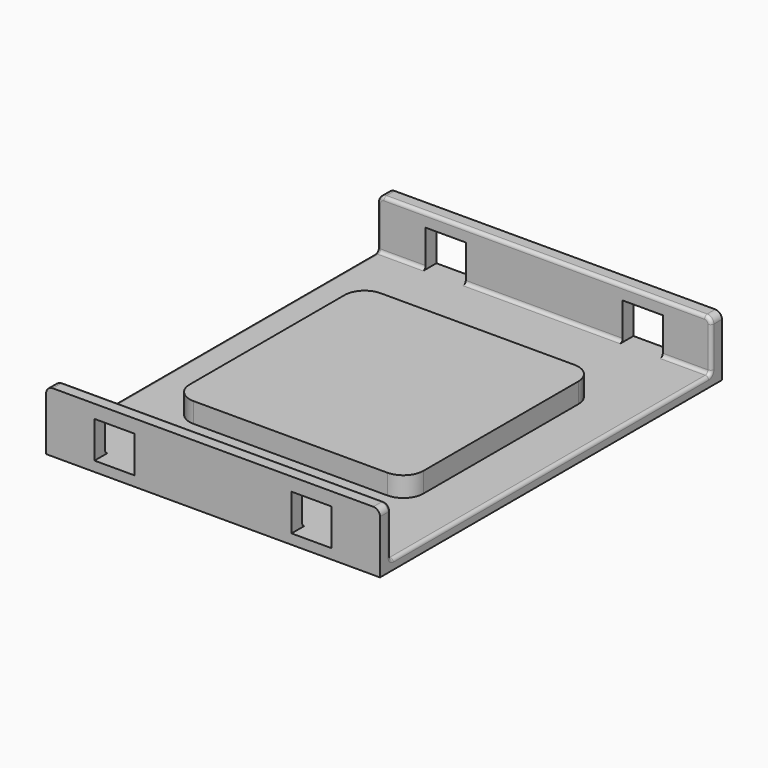
from build123d import *

# Parameters (mm, degrees)
F0_W      = 50
F0_H      = 60
F1_DEPTH  = 1.5
F2_W      = 20
F2_H      = 2
F3_DEPTH  = 9
F4_W      = 6
F4_H      = 5.5
F5_DEPTH  = 32
F6_W      = 35
F6_H      = 35
F7_DEPTH  = 4.5
F8_R      = 3
F9_DEPTH  = 5
F10_DEPTH = 5
F11_DEPTH = 5
F12_DEPTH = 5
F13_R     = 1
F14_R     = 0.5


with BuildPart() as f1:
    # F0 (on Top) → F1 (new body)
    with BuildSketch(Plane.XY):
        Rectangle(F0_W, F0_H)
    extrude(amount=F1_DEPTH)

    # F2 (on Top) → F3 (join)
    with BuildSketch(Plane.XY):
        with Locations((10, 31)):
            Rectangle(F2_W, F2_H)
        with Locations((-10, 31)):
            Rectangle(F2_W, F2_H)
        with Locations((-10, -31)):
            Rectangle(F2_W, F2_H)
        with Locations((10, -31)):
            Rectangle(F2_W, F2_H)
    extrude(amount=F3_DEPTH)

    # F4 (on Front) → F5 (cut, symmetric)
    with BuildSketch(Plane.XZ):
        with Locations((-14.75, 4.25)):
            Rectangle(F4_W, F4_H)
        with Locations((14.75, 4.25)):
            Rectangle(F4_W, F4_H)
    extrude(amount=F5_DEPTH, both=True, mode=Mode.SUBTRACT)

    # F6 (on Top) → F7 (join)
    with BuildSketch(Plane.XY):
        Rectangle(F6_W, F6_H)
    extrude(amount=F7_DEPTH)

    # F8
    f8_edges = [f1.edges().sort_by_distance(p)[0] for p in [
        (17.5, -17.5, 3),
        (-17.5, -17.5, 3),
        (-17.5, 17.5, 3),
        (17.5, 17.5, 3),
    ]]
    fillet(f8_edges, radius=F8_R)

    # F9 (add): a face of the model
    f9_faces = [f1.faces().sort_by_distance(p)[0] for p in [
        (20, -31, 4.5),
    ]]
    extrude(f9_faces, amount=F9_DEPTH)

    # F10 (add): a face of the model
    f10_faces = [f1.faces().sort_by_distance(p)[0] for p in [
        (-20, 31, 4.5),
    ]]
    extrude(f10_faces, amount=F10_DEPTH)

    # F11 (add): a face of the model
    f11_faces = [f1.faces().sort_by_distance(p)[0] for p in [
        (-20, -31, 4.5),
    ]]
    extrude(f11_faces, amount=F11_DEPTH)

    # F12 (add): a face of the model
    f12_faces = [f1.faces().sort_by_distance(p)[0] for p in [
        (20, 31, 4.5),
    ]]
    extrude(f12_faces, amount=F12_DEPTH)

    # F13
    f13_edges = [f1.edges().sort_by_distance(p)[0] for p in [
        (25, 31, 9),
        (-25, -31, 9),
        (-25, 31, 9),
        (25, -31, 9),
    ]]
    fillet(f13_edges, radius=F13_R)

    # F14
    f14_edges = [f1.edges().sort_by_distance(p)[0] for p in [
        (-21.375, 30, 1.5),
        (21.375, 30, 1.5),
        (0, 30, 1.5),
        (-21.375, -30, 1.5),
        (0, -30, 1.5),
        (21.375, -30, 1.5),
        (0, 30, 9),
        (-24.707107, 30, 8.707107),
        (24.707107, 30, 8.707107),
        (-25, 30, 4.75),
        (-25, 0, 1.5),
        (-25, -30, 4.75),
        (25, -30, 4.75),
        (25, 0, 1.5),
        (25, 30, 4.75),
        (-24.707107, -30, 8.707107),
        (0, -30, 9),
        (24.707107, -30, 8.707107),
    ]]
    fillet(f14_edges, radius=F14_R)


solid = f1.part
